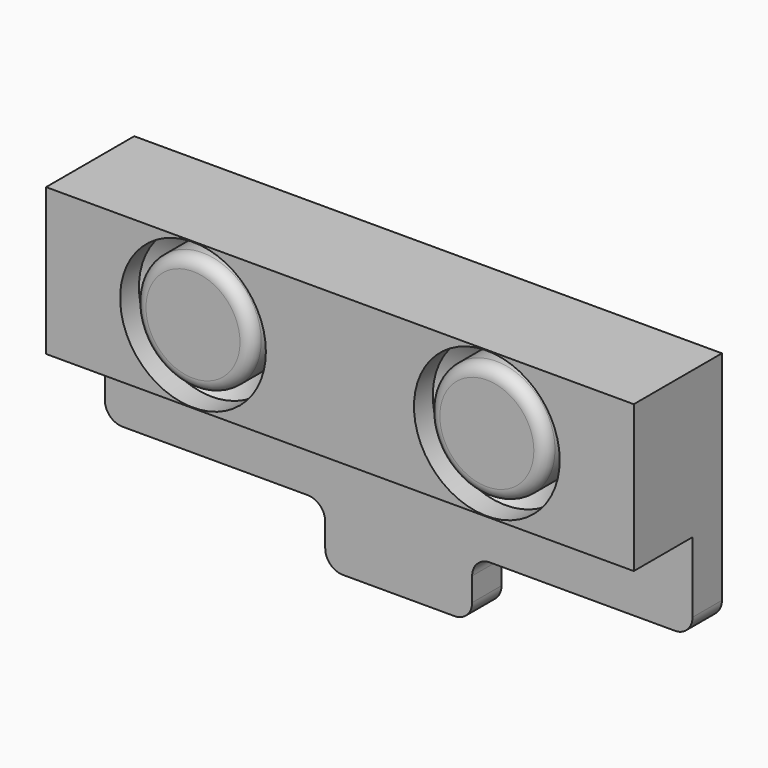
from build123d import *

# Parameters (mm, degrees)
F0_W     = 12.7
F0_H     = 6.35
F1_DEPTH = 0.79375
F2_W     = 4.7625
F2_H     = 1.27
F3_DEPTH = 25.4
F4_R     = 0.381
F2_W_2   = 12.7
F2_H_2   = 3.175
F5_DEPTH = 1.5875
F6_R     = 1.5748
F6_R_2   = 1.27
F7_DEPTH = 0.889
F9_R     = 0.254


# Not quite as in the source:
# - a fillet or chamfer that OpenCascade refuses, or shapes differently, is made with other operations: its cross-section is extruded or revolved along the edge and cut away or added


with BuildPart() as f1:
    # F0 (on Front) → F1 (new body)
    with BuildSketch(Plane.XZ):
        Rectangle(F0_W, F0_H)
    extrude(amount=F1_DEPTH)

    # F2 (on face) → F3 (cut)
    with BuildSketch(Plane.XZ.offset(0.79375)):
        with Locations((-3.96875, -2.54)):
            Rectangle(F2_W, F2_H)
        with Locations((3.96875, -2.54)):
            Rectangle(F2_W, F2_H)
    extrude(amount=-F3_DEPTH, mode=Mode.SUBTRACT)

    # F4
    f4_edges = [f1.edges().sort_by_distance(p)[0] for p in [
        (-1.5875, -0.396875, -3.175),
        (1.5875, -0.396875, -3.175),
        (-6.35, -0.396875, -1.905),
        (6.35, -0.396875, -1.905),
        (1.5875, -0.396875, -1.905),
        (-1.5875, -0.396875, -1.905),
    ]]
    fillet(f4_edges, radius=F4_R)

    # F2 (on face) → F5 (join)
    with BuildSketch(Plane.XZ.offset(0.79375)):
        with Locations((0, 1.5875)):
            Rectangle(F2_W_2, F2_H_2)
    extrude(amount=F5_DEPTH)

    # F6 (on face) → F7 (cut)
    with BuildSketch(Plane.XZ.offset(2.38125)):
        with Locations((-3.175, 1.5875)):
            Circle(F6_R)
        with Locations((-3.175, 1.5875)):
            Circle(F6_R_2, mode=Mode.SUBTRACT)
        with Locations((3.175, 1.5875)):
            Circle(F6_R)
        with Locations((3.175, 1.5875)):
            Circle(F6_R_2, mode=Mode.SUBTRACT)
    extrude(amount=-F7_DEPTH, mode=Mode.SUBTRACT)

    # F8: chamfer of 0.381 on 2 edges, made by hand

    # F8_s1 → F8_t2 (revolve)
    with BuildSketch(Plane.XY.offset(1.5875)):
        Polygon((-1.6002, -1.87325), (-1.9812, -1.49225), (-1.6002, -1.49225), align=None)
    revolve(axis=Axis((-3.175, -1.49225, 1.5875), (0, -1, 0)))

    # F8_s3 → F8_t4 (revolve)
    with BuildSketch(Plane.XY.offset(1.5875)):
        Polygon((4.7498, -1.87325), (4.3688, -1.49225), (4.7498, -1.49225), align=None)
    revolve(axis=Axis((3.175, -1.49225, 1.5875), (0, -1, 0)))

    # F9
    f9_edges = [f1.edges().sort_by_distance(p)[0] for p in [
        (-4.445, -2.38125, 1.5875),
        (1.905, -2.38125, 1.5875),
    ]]
    fillet(f9_edges, radius=F9_R)


solid = f1.part
